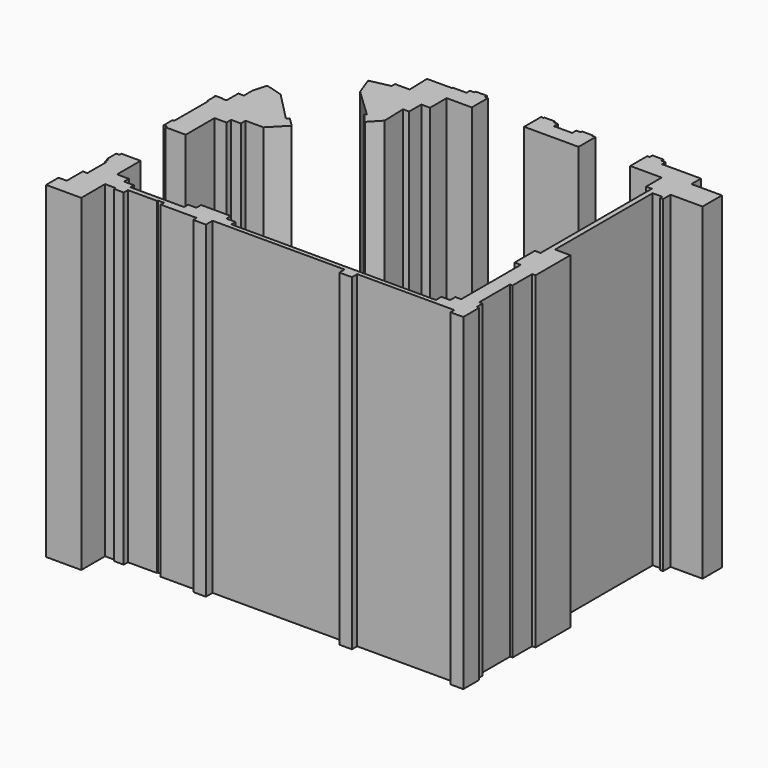
from build123d import *

# Parameters (mm, degrees)
F1_DEPTH = 120
F2_DEPTH = 120
F0_W     = 10
F0_H     = 21.0141725838
F0_W_2   = 19.6411237121
F0_H_2   = 10.4592684656
F0_W_3   = 19.0778486431
F0_H_3   = 10.3107211739
F3_DEPTH = 2


with BuildPart() as f1:
    # F0 (on Top) → F1 (new body)
    with BuildSketch(Plane.XY):
        Polygon((104.0780991316, -23.9835599811), (102.1501421928, -23.9835599811), (102.1501421928, -28.2932731311), (99.9977588654, -28.2932731311), (99.9977588654, -37.7444191278), (102.3042537272, -37.7444191278), (102.3042537272, -65.4667014987), (100.1414619386, -65.4667014987), (100.1414619386, -67.8589488179), (96.8642868102, -67.8589488179), (96.8642868102, -70.4260463626), (58.3577532769, -70.4260463626), (20.6840150058, -70.4260463626), (20.6840150058, -68.4511060626), (17.2706730664, -68.4511060626), (17.2706730664, -66.3842633367), (6.2009952962, -66.3842633367), (6.2009952962, -68.5762241483), (3.1237686053, -68.5762241483), (3.1237686053, -70.4691144983), (-5.4147364572, -70.4691144983), (-16.8841350824, -70.4691144983), (-16.8841350824, -68.8517987728), (-20.4927045852, -68.8517987728), (-20.4927045852, -66.6012912989), (-24.9386969954, -66.6012912989), (-24.9386969954, -55.6243173778), (-32.1035794914, -55.6243173778), (-32.1035794914, -56.4969629049), (-33.2977287471, -56.4969629049), (-33.2977287471, -60.9061233699), (-32.7006541193, -60.9061233699), (-32.7006541193, -62.5595599413), (-32.1954376996, -62.5595599413), (-32.1954376996, -71.3319480419), (-33.8712111115, -71.3319480419), (-33.8712111115, -78.8345783949), (-36.9298607111, -78.8345783949), (-36.9298607111, -84.624171257), (-23.8303467631, -84.624171257), (-23.8303467631, -73.5481083393), (-19.8877826333, -73.5481083393), (-19.8877826333, -74.2829665542), (-16.2919908762, -74.2829665542), (-16.2919908762, -72.3457634449), (-5.4147364572, -72.3457634449), (-5.4147364572, -72.0193969403), (-3.1376881525, -72.0193969403), (-3.1376881525, -73.5192373395), (10.2935563761, -73.5192373395), (10.2935563761, -75.1247169767), (14.9907711882, -75.1247169767), (14.9907711882, -72.0193969403), (64.147684722, -72.0193969403), (64.147684722, -74.4692894016), (68.8449032593, -74.4692894016), (68.8449032593, -72.0193969403), (105.0025410939, -72.0193969403), (105.0025410939, -73.8138692771), (109.7792275238, -73.8138692771), (109.7792275238, -66.4128648434), (108.8904254127, -66.4128648434), (108.8904254127, -63.6571409498), (107.6044253993, -63.6571409498), (107.6044253993, -49.3239933942), (108.5329465556, -49.3239933942), (108.5329465556, -40.2026573513), (109.7792275238, -40.2026573513), (109.7792275238, -23.9835599811), align=None)
        Polygon((99.6696320921, 30.781943351), (99.9977588654, 30.781943351), (99.9977588654, 23.4992671758), (102.1189490928, 23.4992671758), (102.1501421928, 23.4992671758), (102.1501421928, 21.4681793004), (104.0780991316, 21.4681793004), (107.6170546561, 21.4681793004), (107.6170546561, 20.505156368), (108.7368471175, 20.505156368), (108.7368471175, 23.9541213959), (120.6526036038, 23.9541213959), (120.6526036038, 32.972384306), (109.298062101, 32.972384306), (109.298062101, 37.4262184523), (94.853688553, 37.4262184523), (94.853688553, 39.0464030824), (93.2315928489, 39.0464030824), (93.2315928489, 39.9771445118), (89.153733626, 39.9771445118), (89.153733626, 38.6711657047), (88.2695583254, 38.6711657047), (88.2695583254, 30.781943351), align=None)
        Polygon((104.0780991316, 21.4681793004), (102.1501421928, 21.4681793004), (102.1501421928, 8.9439952115), (102.1501421928, -23.9835599811), (104.0780991316, -23.9835599811), align=None)
    extrude(amount=F1_DEPTH)

    # F0 (on Top) → F3 (join)
    with BuildSketch(Plane.XY):
        Polygon((99.6696320921, 30.781943351), (99.9977588654, 30.781943351), (99.9977588654, 23.4992671758), (102.1189490928, 23.4992671758), (102.1501421928, 23.4992671758), (102.1501421928, 21.4681793004), (104.0780991316, 21.4681793004), (107.6170546561, 21.4681793004), (107.6170546561, 20.505156368), (108.7368471175, 20.505156368), (108.7368471175, 23.9541213959), (120.6526036038, 23.9541213959), (120.6526036038, 32.972384306), (109.298062101, 32.972384306), (109.298062101, 37.4262184523), (94.853688553, 37.4262184523), (94.853688553, 39.0464030824), (93.2315928489, 39.0464030824), (93.2315928489, 39.9771445118), (89.153733626, 39.9771445118), (89.153733626, 38.6711657047), (88.2695583254, 38.6711657047), (88.2695583254, 30.781943351), align=None)
        with BuildLine():
            Line((99.6696320921, 23.4992671758), (99.6696320921, 30.781943351))
            Line((99.6696320921, 30.781943351), (88.2695583254, 30.781943351))
            Line((88.2695583254, 30.781943351), (69.0153879672, 30.781943351))
            Line((69.0153879672, 30.781943351), (48.762787655, 30.781943351))
            Line((48.762787655, 30.781943351), (29.2577525228, 30.781943351))
            Line((29.2577525228, 30.781943351), (19.9045134336, 30.781943351))
            Line((19.9045134336, 30.781943351), (19.9045134336, 23.0269022286))
            Line((19.9045134336, 23.0269022286), (16.6568593681, 23.0269022286))
            Line((16.6568593681, 23.0269022286), (16.6568593681, 17.3791721463))
            Line((16.6568593681, 17.3791721463), (14.3733127043, 17.3791721463))
            Line((14.3733127043, 17.3791721463), (14.6709829569, 8.4714386612))
            Line((14.6709829569, 8.4714386612), (10.6844678521, 4.2303507216))
            Line((10.6844678521, 4.2303507216), (-4.4199563004, -10.9154852107))
            Line((-4.4199563004, -10.9154852107), (-10.2235677003, -16.8631691486))
            Line((-10.2235677003, -16.8631691486), (-16.8841350824, -16.8631691486))
            Line((-16.8841350824, -16.8631691486), (-16.8841350824, -19.0303940326))
            Line((-16.8841350824, -19.0303940326), (-20.4927045852, -19.0303940326))
            Line((-20.4927045852, -19.0303940326), (-20.4927045852, -21.2057642639))
            Line((-20.4927045852, -21.2057642639), (-24.9386969954, -21.2057642639))
            Line((-24.9386969954, -21.2057642639), (-24.9386969954, -34.610144794))
            Line((-24.9386969954, -34.610144794), (-24.9386969954, -55.6243173778))
            Line((-24.9386969954, -55.6243173778), (-24.9386969954, -66.6012912989))
            Line((-24.9386969954, -66.6012912989), (-20.4927045852, -66.6012912989))
            Line((-20.4927045852, -66.6012912989), (-20.4927045852, -68.8517987728))
            Line((-20.4927045852, -68.8517987728), (-16.8841350824, -68.8517987728))
            Line((-16.8841350824, -68.8517987728), (-16.8841350824, -70.4691144983))
            Line((-16.8841350824, -70.4691144983), (-5.4147364572, -70.4691144983))
            add(Edge.make_bspline(
                [(102.1501421928, 8.9439952115), (96.4144905089, 9.5971060874), (74.7102468697, 6.7231432238), (66.3654978969, -13.0116481431), (57.312284926, -42.0365016133), (23.6452919147, -36.9521370841), (-0.5289780071, -50.1700454327), (-5.3005459083, -59.2095740287), (-5.4147364572, -70.4691144983)],
                knots=[0, 0, 0, 0, 0.1666919347, 0.3217482447, 0.4926564614, 0.6771110907, 0.8451990117, 1, 1, 1, 1], degree=3))
            Line((102.1501421928, 8.9439952115), (102.1501421928, 21.4681793004))
            Line((102.1501421928, 21.4681793004), (102.1189490928, 21.4681793004))
            Line((102.1189490928, 21.4681793004), (102.1189490928, 23.4992671758))
            Line((102.1189490928, 23.4992671758), (99.9977588654, 23.4992671758))
            Line((99.9977588654, 23.4992671758), (99.6696320921, 23.4992671758))
        make_face()
        with Locations((-17.4386969954, -45.1172310859)):
            Rectangle(F0_W, F0_H, mode=Mode.SUBTRACT)
        Polygon((29.6495072544, 28.281943351), (48.7273558974, 28.281943351), (48.7273558974, 28.1333960593), (48.7273558974, 17.8226748854), (29.6495072544, 17.8226748854), (29.6495072544, 28.1333960593), align=None, mode=Mode.SUBTRACT)
        with Locations((78.77965644, 23.0523091182)):
            Rectangle(F0_W_2, F0_H_2, mode=Mode.SUBTRACT)
        Polygon((48.762787655, 30.781943351), (69.0153879672, 30.781943351), (69.0153879672, 38.6711657047), (67.7313586324, 38.6711657047), (67.7313586324, 39.0001275263), (63.7430814654, 39.0001275263), (63.7430814654, 38.3571237944), (62.0821272582, 38.3571237944), (62.0821272582, 36.4718586206), (55.2846682817, 36.4718586206), (55.2846682817, 38.3571237944), (53.7230936438, 38.3571237944), (53.7230936438, 39.0001275263), (49.6813622862, 39.0001275263), (49.6813622862, 38.6711657047), (48.762787655, 38.6711657047), align=None)
        Polygon((104.0780991316, 21.4681793004), (102.1501421928, 21.4681793004), (102.1501421928, 8.9439952115), (102.1501421928, -23.9835599811), (104.0780991316, -23.9835599811), align=None)
        Polygon((19.9045134336, 30.781943351), (29.2577525228, 30.781943351), (29.2577525228, 38.2338815712), (28.1164560237, 38.2338815712), (28.1164560237, 39.2731332564), (23.9018283554, 39.2731332564), (23.9018283554, 38.644535222), (22.2943208881, 38.644535222), (22.2943208881, 37.03703148), (17.1962294497, 37.03703148), (17.1962294497, 36.692565062), (7.8619390496, 36.692565062), (8.1207575276, 28.3034723252), (2.6483471133, 28.3034723252), (2.6483471133, 26.7531967218), (-4.8212543502, 25.1207724214), (-2.288084887, 18.2357467711), (8.1207575276, 8.3491299301), (7.5900321826, 7.7588022687), (10.6844678521, 4.2303507216), (14.6709829569, 8.4714386612), (14.3733127043, 17.3791721463), (16.6568593681, 17.3791721463), (16.6568593681, 23.0269022286), (19.9045134336, 23.0269022286), align=None)
        Polygon((104.0780991316, -23.9835599811), (102.1501421928, -23.9835599811), (102.1501421928, -28.2932731311), (99.9977588654, -28.2932731311), (99.9977588654, -37.7444191278), (102.3042537272, -37.7444191278), (102.3042537272, -65.4667014987), (100.1414619386, -65.4667014987), (100.1414619386, -67.8589488179), (96.8642868102, -67.8589488179), (96.8642868102, -70.4260463626), (58.3577532769, -70.4260463626), (20.6840150058, -70.4260463626), (20.6840150058, -68.4511060626), (17.2706730664, -68.4511060626), (17.2706730664, -66.3842633367), (6.2009952962, -66.3842633367), (6.2009952962, -68.5762241483), (3.1237686053, -68.5762241483), (3.1237686053, -70.4691144983), (-5.4147364572, -70.4691144983), (-16.8841350824, -70.4691144983), (-16.8841350824, -68.8517987728), (-20.4927045852, -68.8517987728), (-20.4927045852, -66.6012912989), (-24.9386969954, -66.6012912989), (-24.9386969954, -55.6243173778), (-32.1035794914, -55.6243173778), (-32.1035794914, -56.4969629049), (-33.2977287471, -56.4969629049), (-33.2977287471, -60.9061233699), (-32.7006541193, -60.9061233699), (-32.7006541193, -62.5595599413), (-32.1954376996, -62.5595599413), (-32.1954376996, -71.3319480419), (-33.8712111115, -71.3319480419), (-33.8712111115, -78.8345783949), (-36.9298607111, -78.8345783949), (-36.9298607111, -84.624171257), (-23.8303467631, -84.624171257), (-23.8303467631, -73.5481083393), (-19.8877826333, -73.5481083393), (-19.8877826333, -74.2829665542), (-16.2919908762, -74.2829665542), (-16.2919908762, -72.3457634449), (-5.4147364572, -72.3457634449), (-5.4147364572, -72.0193969403), (-3.1376881525, -72.0193969403), (-3.1376881525, -73.5192373395), (10.2935563761, -73.5192373395), (10.2935563761, -75.1247169767), (14.9907711882, -75.1247169767), (14.9907711882, -72.0193969403), (64.147684722, -72.0193969403), (64.147684722, -74.4692894016), (68.8449032593, -74.4692894016), (68.8449032593, -72.0193969403), (105.0025410939, -72.0193969403), (105.0025410939, -73.8138692771), (109.7792275238, -73.8138692771), (109.7792275238, -66.4128648434), (108.8904254127, -66.4128648434), (108.8904254127, -63.6571409498), (107.6044253993, -63.6571409498), (107.6044253993, -49.3239933942), (108.5329465556, -49.3239933942), (108.5329465556, -40.2026573513), (109.7792275238, -40.2026573513), (109.7792275238, -23.9835599811), align=None)
        Polygon((-4.4199563004, -10.9154852107), (10.6844678521, 4.2303507216), (7.5900321826, 7.7588022687), (8.1207575276, 8.3491299301), (-2.288084887, 18.2357467711), (-4.8212543502, 25.1207724214), (-25.6785540283, 4.3204217218), (-19.305137941, 2.4789126496), (-8.6173633486, -8.3917845041), (-7.7413897403, -7.6712942682), align=None)
        Polygon((-10.2235677003, -16.8631691486), (-4.4199563004, -10.9154852107), (-7.7413897403, -7.6712942682), (-8.6173633486, -8.3917845041), (-19.305137941, 2.4789126496), (-25.6785540283, 4.3204217218), (-27.1482723206, -0.7662359276), (-27.1482723206, -4.8009688035), (-29.216985628, -4.8009688035), (-29.216985628, -10.270296596), (-30.7166962326, -10.270296596), (-30.7166962326, -10.0897120821), (-33.6742246896, -10.0897120821), (-33.6742246896, -10.270296596), (-33.3715299517, -10.270296596), (-33.3715299517, -13.8538731262), (-33.0317016242, -13.8538731262), (-33.0317016242, -29.7705680132), (-33.6742246896, -29.7705680132), (-33.6742246896, -33.9439176023), (-32.3900463432, -33.9439176023), (-32.3900463432, -34.610144794), (-24.9386969954, -34.610144794), (-24.9386969954, -21.2057642639), (-20.4927045852, -21.2057642639), (-20.4927045852, -19.0303940326), (-16.8841350824, -19.0303940326), (-16.8841350824, -16.8631691486), align=None)
        with Locations((-17.4386969954, -45.1172310859)):
            Rectangle(F0_W, F0_H)
        with BuildLine():
            Line((102.1501421928, -23.9835599811), (102.1501421928, 8.9439952115))
            add(Edge.make_bspline(
                [(102.1501421928, 8.9439952115), (96.4144905089, 9.5971060874), (74.7102468697, 6.7231432238), (66.3654978969, -13.0116481431), (57.312284926, -42.0365016133), (23.6452919147, -36.9521370841), (-0.5289780071, -50.1700454327), (-5.3005459083, -59.2095740287), (-5.4147364572, -70.4691144983)],
                knots=[0, 0, 0, 0, 0.1666919347, 0.3217482447, 0.4926564614, 0.6771110907, 0.8451990117, 1, 1, 1, 1], degree=3))
            Line((-5.4147364572, -70.4691144983), (3.1237686053, -70.4691144983))
            Line((3.1237686053, -70.4691144983), (3.1237686053, -68.5762241483))
            Line((3.1237686053, -68.5762241483), (6.2009952962, -68.5762241483))
            Line((6.2009952962, -68.5762241483), (6.2009952962, -66.3842633367))
            Line((6.2009952962, -66.3842633367), (17.2706730664, -66.3842633367))
            Line((17.2706730664, -66.3842633367), (17.2706730664, -68.4511060626))
            Line((17.2706730664, -68.4511060626), (20.6840150058, -68.4511060626))
            Line((20.6840150058, -68.4511060626), (20.6840150058, -70.4260463626))
            Line((20.6840150058, -70.4260463626), (58.3577532769, -70.4260463626))
            ThreePointArc((58.3577532769, -70.4260463626), (70.3790964817, -40.6639056729), (99.9977588654, -28.2932731311))
            Line((99.9977588654, -28.2932731311), (102.1501421928, -28.2932731311))
            Line((102.1501421928, -28.2932731311), (102.1501421928, -23.9835599811))
        make_face()
        with BuildLine():
            Line((99.9977588654, -37.7444191278), (99.9977588654, -28.2932731311))
            ThreePointArc((99.9977588654, -28.2932731311), (70.3790964817, -40.6639056729), (58.3577532769, -70.4260463626))
            Line((58.3577532769, -70.4260463626), (96.8642868102, -70.4260463626))
            Line((96.8642868102, -70.4260463626), (96.8642868102, -67.8589488179))
            Line((96.8642868102, -67.8589488179), (100.1414619386, -67.8589488179))
            Line((100.1414619386, -67.8589488179), (100.1414619386, -65.4667014987))
            Line((100.1414619386, -65.4667014987), (102.3042537272, -65.4667014987))
            Line((102.3042537272, -65.4667014987), (102.3042537272, -37.7444191278))
            Line((102.3042537272, -37.7444191278), (99.9977588654, -37.7444191278))
        make_face()
        with Locations((78.77965644, 23.0523091182)):
            Rectangle(F0_W_2, F0_H_2)
        with Locations((39.1884315759, 22.9780354723)):
            Rectangle(F0_W_3, F0_H_3)
    extrude(amount=-F3_DEPTH)


with BuildPart() as f2:
    # F0 (on Top) → F2 (new body)
    with BuildSketch(Plane.XY):
        Polygon((48.762787655, 30.781943351), (69.0153879672, 30.781943351), (69.0153879672, 38.6711657047), (67.7313586324, 38.6711657047), (67.7313586324, 39.0001275263), (63.7430814654, 39.0001275263), (63.7430814654, 38.3571237944), (62.0821272582, 38.3571237944), (62.0821272582, 36.4718586206), (55.2846682817, 36.4718586206), (55.2846682817, 38.3571237944), (53.7230936438, 38.3571237944), (53.7230936438, 39.0001275263), (49.6813622862, 39.0001275263), (49.6813622862, 38.6711657047), (48.762787655, 38.6711657047), align=None)
    extrude(amount=F2_DEPTH)


with BuildPart() as f2b:
    # F0 (on Top) → F2, piece 2 (new body)
    with BuildSketch(Plane.XY):
        Polygon((19.9045134336, 30.781943351), (29.2577525228, 30.781943351), (29.2577525228, 38.2338815712), (28.1164560237, 38.2338815712), (28.1164560237, 39.2731332564), (23.9018283554, 39.2731332564), (23.9018283554, 38.644535222), (22.2943208881, 38.644535222), (22.2943208881, 37.03703148), (17.1962294497, 37.03703148), (17.1962294497, 36.692565062), (7.8619390496, 36.692565062), (8.1207575276, 28.3034723252), (2.6483471133, 28.3034723252), (2.6483471133, 26.7531967218), (-4.8212543502, 25.1207724214), (-2.288084887, 18.2357467711), (8.1207575276, 8.3491299301), (7.5900321826, 7.7588022687), (10.6844678521, 4.2303507216), (14.6709829569, 8.4714386612), (14.3733127043, 17.3791721463), (16.6568593681, 17.3791721463), (16.6568593681, 23.0269022286), (19.9045134336, 23.0269022286), align=None)
    extrude(amount=F2_DEPTH)


with BuildPart() as f2c:
    # F0 (on Top) → F2, piece 3 (new body)
    with BuildSketch(Plane.XY):
        Polygon((-10.2235677003, -16.8631691486), (-4.4199563004, -10.9154852107), (-7.7413897403, -7.6712942682), (-8.6173633486, -8.3917845041), (-19.305137941, 2.4789126496), (-25.6785540283, 4.3204217218), (-27.1482723206, -0.7662359276), (-27.1482723206, -4.8009688035), (-29.216985628, -4.8009688035), (-29.216985628, -10.270296596), (-30.7166962326, -10.270296596), (-30.7166962326, -10.0897120821), (-33.6742246896, -10.0897120821), (-33.6742246896, -10.270296596), (-33.3715299517, -10.270296596), (-33.3715299517, -13.8538731262), (-33.0317016242, -13.8538731262), (-33.0317016242, -29.7705680132), (-33.6742246896, -29.7705680132), (-33.6742246896, -33.9439176023), (-32.3900463432, -33.9439176023), (-32.3900463432, -34.610144794), (-24.9386969954, -34.610144794), (-24.9386969954, -21.2057642639), (-20.4927045852, -21.2057642639), (-20.4927045852, -19.0303940326), (-16.8841350824, -19.0303940326), (-16.8841350824, -16.8631691486), align=None)
    extrude(amount=F2_DEPTH)


solid = Compound([f1.part, f2.part, f2b.part, f2c.part])
